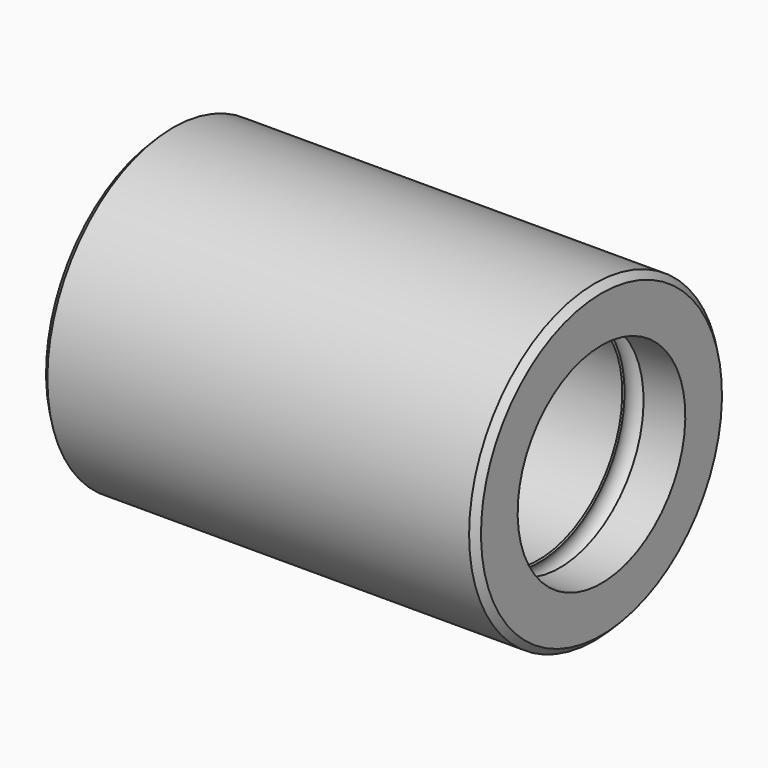
from build123d import *

# Parameters (mm, degrees)
F2_SIZE = 1.6002


# Not quite as in the source:
# - a fillet or chamfer that OpenCascade refuses, or shapes differently, is made with other operations: its cross-section is extruded or revolved along the edge and cut away or added


with BuildPart() as f1:
    # F0 (on Front) → F1 (revolve)
    with BuildSketch(Plane.XZ):
        with BuildLine():
            Line((0.0191729553, 38.0993708088), (-105.3908270447, 38.0993708088))
            Line((-105.3908270447, 38.0993708088), (-105.3908270447, 25.3993708088))
            Line((-105.3908270447, 25.3993708088), (-94.5958270447, 25.3993708088))
            ThreePointArc((-94.5958270447, 25.3993708088), (-92.6908270447, 31.1143708088), (-90.7858270447, 25.3993708088))
            Line((-90.7858270447, 25.3993708088), (-14.5858270447, 25.3993708088))
            ThreePointArc((-14.5858270447, 25.3993708088), (-12.6808270447, 31.1143708088), (-10.7758270447, 25.3993708088))
            Line((-10.7758270447, 25.3993708088), (0.0191729553, 25.3993708088))
            Line((0.0191729553, 25.3993708088), (0.0191729553, 38.0993708088))
        make_face()
    revolve(axis=Axis((-52.7064110639, 0, -0.0006291912), (1, 0, 0)))

    # F2
    f2_edges = [f1.edges().sort_by_distance(p)[0] for p in [
        (-105.390827, 0, -38.100629),
        (0.019173, 0, -38.100629),
    ]]
    chamfer(f2_edges, length=F2_SIZE)

    # F3: chamfer of 0.79375 on 4 edges, made by hand

    # F3_s1 → F3_t2 (revolve, cut)
    with BuildSketch(Plane.XZ):
        with BuildLine():
            Line((-10.0883836418, 25.3704317814), (-10.3129200756, 25.8679252209))
            Line((-10.3129200756, 25.8679252209), (-10.3248249165, 25.8784271439))
            ThreePointArc((-10.3248249165, 25.8784271439), (-10.5336671168, 25.6220933094), (-10.7853520447, 25.4120708088))
            Line((-10.7853520447, 25.4120708088), (-10.7758270447, 25.3834958088))
            ThreePointArc((-10.7758270447, 25.3834958088), (-10.4321053433, 25.3834958088), (-10.0883836418, 25.3545567814))
            Line((-10.0883836418, 25.3545567814), (-10.0883836418, 25.3704317814))
        make_face()
    revolve(axis=Axis((-10.7758270447, 0, -0.0006291912), (1, 0, 0)), mode=Mode.SUBTRACT)

    # F3_s3 → F3_t4 (revolve, cut)
    with BuildSketch(Plane.XZ):
        with BuildLine():
            Line((-15.0487340139, 25.8679252209), (-15.2732704477, 25.3704317814))
            Line((-15.2732704477, 25.3704317814), (-15.2732704477, 25.3545567814))
            ThreePointArc((-15.2732704477, 25.3545567814), (-14.9295487462, 25.3834958088), (-14.5858270447, 25.3834958088))
            Line((-14.5858270447, 25.3834958088), (-14.5763020447, 25.4120708088))
            ThreePointArc((-14.5763020447, 25.4120708088), (-14.8279869727, 25.6220933094), (-15.036829173, 25.8784271439))
            Line((-15.036829173, 25.8784271439), (-15.0487340139, 25.8679252209))
        make_face()
    revolve(axis=Axis((-14.5858270447, 0, -0.0006291912), (1, 0, 0)), mode=Mode.SUBTRACT)

    # F3_s5 → F3_t6 (revolve, cut)
    with BuildSketch(Plane.XZ):
        with BuildLine():
            Line((-90.0983836418, 25.3704317814), (-90.3229200756, 25.8679252209))
            Line((-90.3229200756, 25.8679252209), (-90.3348249165, 25.8784271439))
            ThreePointArc((-90.3348249165, 25.8784271439), (-90.5436671168, 25.6220933094), (-90.7953520447, 25.4120708088))
            Line((-90.7953520447, 25.4120708088), (-90.7858270447, 25.3834958088))
            ThreePointArc((-90.7858270447, 25.3834958088), (-90.4421053433, 25.3834958088), (-90.0983836418, 25.3545567814))
            Line((-90.0983836418, 25.3545567814), (-90.0983836418, 25.3704317814))
        make_face()
    revolve(axis=Axis((-90.7858270447, 0, -0.0006291912), (1, 0, 0)), mode=Mode.SUBTRACT)

    # F3_s7 → F3_t8 (revolve, cut)
    with BuildSketch(Plane.XZ):
        with BuildLine():
            Line((-95.0587340139, 25.8679252209), (-95.2832704477, 25.3704317814))
            Line((-95.2832704477, 25.3704317814), (-95.2832704477, 25.3545567814))
            ThreePointArc((-95.2832704477, 25.3545567814), (-94.9395487462, 25.3834958088), (-94.5958270447, 25.3834958088))
            Line((-94.5958270447, 25.3834958088), (-94.5863020447, 25.4120708088))
            ThreePointArc((-94.5863020447, 25.4120708088), (-94.8379869727, 25.6220933094), (-95.046829173, 25.8784271439))
            Line((-95.046829173, 25.8784271439), (-95.0587340139, 25.8679252209))
        make_face()
    revolve(axis=Axis((-94.5958270447, 0, -0.0006291912), (1, 0, 0)), mode=Mode.SUBTRACT)


solid = f1.part
